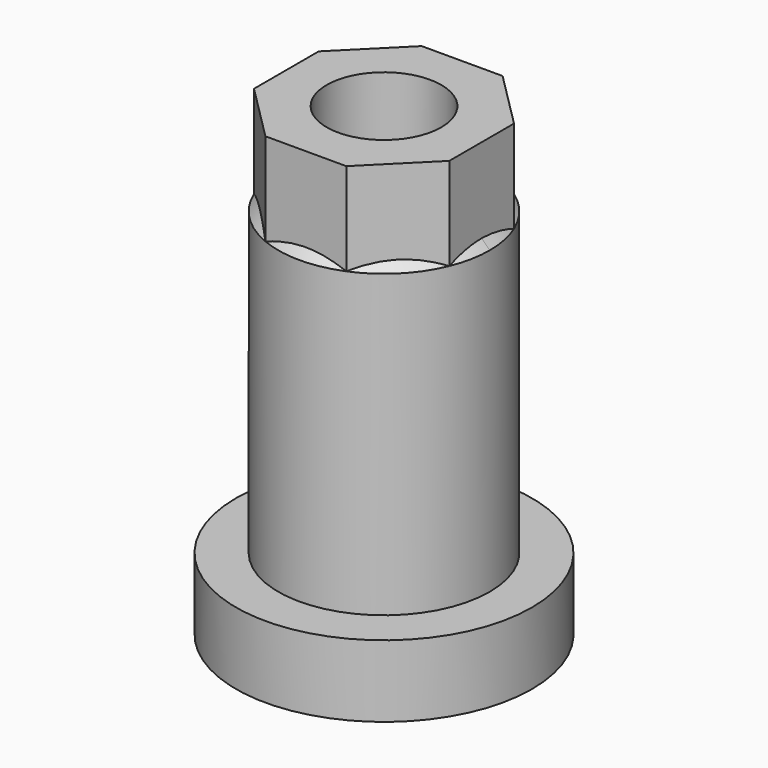
from build123d import *

# Parameters (mm, degrees)
F0_R         = 5.55625
F0_R_2       = 2.15265
F1_DEPTH     = 2.69875
F2_R         = 3.96875
F2_R_2       = 2.15265
F3_DEPTH     = 11.58875
F4_R         = 2.15265
F5_DEPTH     = 3.175
F6_T4_ANGLE  = 45
F6_T9_ANGLE  = 45
F6_T14_ANGLE = 45
F6_T19_ANGLE = 45
F6_T24_ANGLE = 45
F6_T29_ANGLE = 45
F6_T34_ANGLE = 45
F6_T39_ANGLE = 22.5
F6_T44_ANGLE = 22.5


# Not quite as in the source:
# - a fillet or chamfer that OpenCascade refuses, or shapes differently, is made with other operations: its cross-section is extruded or revolved along the edge and cut away or added


with BuildPart() as f1:
    # F0 (on Top) → F1 (new body)
    with BuildSketch(Plane.XY):
        Circle(F0_R)
        Circle(F0_R_2, mode=Mode.SUBTRACT)
    extrude(amount=F1_DEPTH)

    # F2 (on face) → F3 (join)
    with BuildSketch(Plane.XY.offset(2.69875)):
        Circle(F2_R)
        Circle(F2_R_2, mode=Mode.SUBTRACT)
    extrude(amount=F3_DEPTH)

    # F4 (on face) → F5 (join)
    with BuildSketch(Plane.XY.offset(14.2875)):
        Polygon((-3.6666468947, 1.5187748722), (-3.6666468947, -1.5187748722), (-1.5187748722, -3.6666468947), (1.5187748722, -3.6666468947), (3.6666468947, -1.5187748722), (3.6666468947, 1.5187748722), (1.5187748722, 3.6666468947), (-1.5187748722, 3.6666468947), align=None)
        Circle(F4_R, mode=Mode.SUBTRACT)
    extrude(amount=F5_DEPTH)

    # F6: chamfer of 0.3021076 on 7 edges, made by hand


with BuildPart() as f6_tool2:
    # F6_s3 → F6_t4 (revolve)
    with BuildSketch(Plane(origin=(0, 0, 0), x_dir=(0, 0, 1), z_dir=(0.3826834324, 0.9238795325, 0))):
        Polygon((13.9853924, -3.96875), (14.2875, -3.6666424), (14.2875, -3.96875), align=None)
    revolve(axis=Axis((0, 0, 14.2875), (0, 0, 1)), revolution_arc=F6_T4_ANGLE)

    split(bisect_by=Plane.YZ.offset(-3.6666468947), keep=Keep.BOTTOM)


with BuildPart() as f1_1:
    add(f1.part)

    # F6_t1: cut F6_tool2
    add(f6_tool2.part, mode=Mode.SUBTRACT)


with BuildPart() as f6_tool7:
    # F6_s8 → F6_t9 (revolve)
    with BuildSketch(Plane(origin=(0, 0, 0), x_dir=(0, 0, 1), z_dir=(0.9238795325, 0.3826834324, 0))):
        Polygon((13.9853924, -3.96875), (14.2875, -3.6666424), (14.2875, -3.96875), align=None)
    revolve(axis=Axis((0, 0, 14.2875), (0, 0, 1)), revolution_arc=F6_T9_ANGLE)

    split(bisect_by=Plane(origin=(-2.5927108834, 2.5927108834, 0), x_dir=(0, 0, 1), z_dir=(-0.7071067812, 0.7071067812, 0)), keep=Keep.TOP)


with BuildPart() as f1_2:
    add(f1_1.part)

    # F6_t6: cut F6_tool7
    add(f6_tool7.part, mode=Mode.SUBTRACT)


with BuildPart() as f6_tool12:
    # F6_s13 → F6_t14 (revolve)
    with BuildSketch(Plane(origin=(0, 0, 0), x_dir=(0, 0, 1), z_dir=(0.9238795325, -0.3826834324, 0))):
        Polygon((13.9853924, -3.96875), (14.2875, -3.6666424), (14.2875, -3.96875), align=None)
    revolve(axis=Axis((0, 0, 14.2875), (0, 0, 1)), revolution_arc=F6_T14_ANGLE)

    split(bisect_by=Plane.XZ.offset(-3.6666468947), keep=Keep.BOTTOM)


with BuildPart() as f1_3:
    add(f1_2.part)

    # F6_t11: cut F6_tool12
    add(f6_tool12.part, mode=Mode.SUBTRACT)


with BuildPart() as f6_tool17:
    # F6_s18 → F6_t19 (revolve)
    with BuildSketch(Plane(origin=(0, 0, 0), x_dir=(0, 0, 1), z_dir=(0.3826834324, -0.9238795325, 0))):
        Polygon((13.9853924, -3.96875), (14.2875, -3.6666424), (14.2875, -3.96875), align=None)
    revolve(axis=Axis((0, 0, 14.2875), (0, 0, 1)), revolution_arc=F6_T19_ANGLE)

    split(bisect_by=Plane(origin=(2.5927108834, 2.5927108834, 0), x_dir=(0, 0, 1), z_dir=(0.7071067812, 0.7071067812, 0)), keep=Keep.TOP)


with BuildPart() as f1_4:
    add(f1_3.part)

    # F6_t16: cut F6_tool17
    add(f6_tool17.part, mode=Mode.SUBTRACT)


with BuildPart() as f6_tool22:
    # F6_s23 → F6_t24 (revolve)
    with BuildSketch(Plane(origin=(0, 0, 0), x_dir=(0, 0, 1), z_dir=(-0.9238795325, -0.3826834324, 0))):
        Polygon((13.9853924, -3.96875), (14.2875, -3.6666424), (14.2875, -3.96875), align=None)
    revolve(axis=Axis((0, 0, 14.2875), (0, 0, 1)), revolution_arc=F6_T24_ANGLE)

    split(bisect_by=Plane(origin=(2.5927108834, -2.5927108834, 0), x_dir=(0, 0, 1), z_dir=(0.7071067812, -0.7071067812, 0)), keep=Keep.TOP)


with BuildPart() as f1_5:
    add(f1_4.part)

    # F6_t21: cut F6_tool22
    add(f6_tool22.part, mode=Mode.SUBTRACT)


with BuildPart() as f6_tool27:
    # F6_s28 → F6_t29 (revolve)
    with BuildSketch(Plane(origin=(0, 0, 0), x_dir=(0, 0, 1), z_dir=(-0.9238795325, 0.3826834324, 0))):
        Polygon((13.9853924, -3.96875), (14.2875, -3.6666424), (14.2875, -3.96875), align=None)
    revolve(axis=Axis((0, 0, 14.2875), (0, 0, 1)), revolution_arc=F6_T29_ANGLE)

    split(bisect_by=Plane.XZ.offset(3.6666468947), keep=Keep.TOP)


with BuildPart() as f1_6:
    add(f1_5.part)

    # F6_t26: cut F6_tool27
    add(f6_tool27.part, mode=Mode.SUBTRACT)


with BuildPart() as f6_tool32:
    # F6_s33 → F6_t34 (revolve)
    with BuildSketch(Plane(origin=(0, 0, 0), x_dir=(0, 0, 1), z_dir=(-0.3826834324, 0.9238795325, 0))):
        Polygon((13.9853924, -3.96875), (14.2875, -3.6666424), (14.2875, -3.96875), align=None)
    revolve(axis=Axis((0, 0, 14.2875), (0, 0, 1)), revolution_arc=F6_T34_ANGLE)

    split(bisect_by=Plane(origin=(-2.5927108834, -2.5927108834, 0), x_dir=(0, 0, 1), z_dir=(-0.7071067812, -0.7071067812, 0)), keep=Keep.TOP)


with BuildPart() as f1_7:
    add(f1_6.part)

    # F6_t31: cut F6_tool32
    add(f6_tool32.part, mode=Mode.SUBTRACT)


with BuildPart() as f6_tool37:
    # F6_s38 → F6_t39 (revolve)
    with BuildSketch(Plane(origin=(0, 0, 0), x_dir=(0, 0, 1), z_dir=(-0.3826834324, -0.9238795325, 0))):
        Polygon((13.9853924, -3.96875), (14.2875, -3.6666424), (14.2875, -3.96875), align=None)
    revolve(axis=Axis((0, 0, 14.2875), (0, 0, 1)), revolution_arc=F6_T39_ANGLE)

    split(bisect_by=Plane.YZ.offset(3.6666468947), keep=Keep.TOP)


with BuildPart() as f1_8:
    add(f1_7.part)

    # F6_t36: cut F6_tool37
    add(f6_tool37.part, mode=Mode.SUBTRACT)


with BuildPart() as f6_tool42:
    # F6_s43 → F6_t44 (revolve)
    with BuildSketch(Plane.XZ):
        Polygon((3.96875, 13.9853924), (3.6666424, 14.2875), (3.96875, 14.2875), align=None)
    revolve(axis=Axis((0, 0, 14.2875), (0, 0, 1)), revolution_arc=F6_T44_ANGLE)

    split(bisect_by=Plane.YZ.offset(3.6666468947), keep=Keep.TOP)


with BuildPart() as f1_9:
    add(f1_8.part)

    # F6_t41: cut F6_tool42
    add(f6_tool42.part, mode=Mode.SUBTRACT)


solid = f1_9.part
